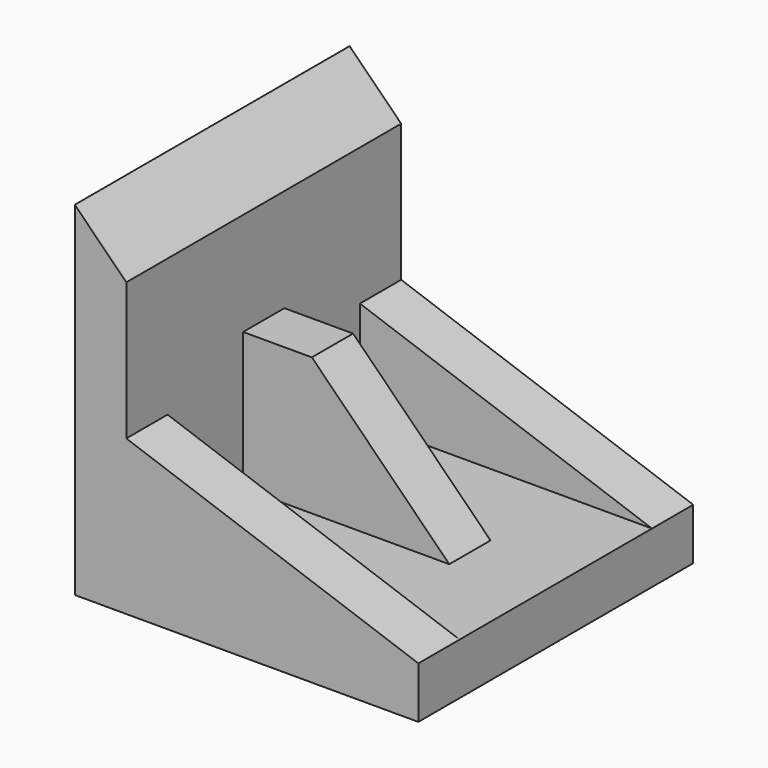
from build123d import *

# Parameters (mm, degrees)
F1_DEPTH = 127
F3_DEPTH = 38.1
F4_DEPTH = 19.05


# Not quite as in the source:
# - a pattern or mirror of a feature is missing from the dataset's text; its kind, count and spacing are read off the source's solid


with BuildPart() as f1:
    # F0 (on Front) → F1 (new body, symmetric)
    with BuildSketch(Plane.XZ):
        Polygon((0, 254), (0, 0), (254, 0), (254, 38.1), (190.5, 38.1), (38.1, 38.1), (38.1, 139.7), (38.1, 215.9), align=None)
    extrude(amount=F1_DEPTH, both=True)

    # F2 (on face) → F3 (join)
    with BuildSketch(Plane.XZ.offset(127)):
        Polygon((254, 38.1), (38.1, 114.3), (38.1, 38.1), align=None)
    f3 = extrude(amount=-F3_DEPTH)

    # F3_copies: F3 across plane
    add(f3.mirror(Plane.ZX))

    # F0 (on Front) → F4 (join, symmetric)
    with BuildSketch(Plane.XZ):
        Polygon((38.1, 38.1), (190.5, 38.1), (88.9, 139.7), (38.1, 139.7), align=None)
    extrude(amount=F4_DEPTH, both=True)


solid = f1.part
